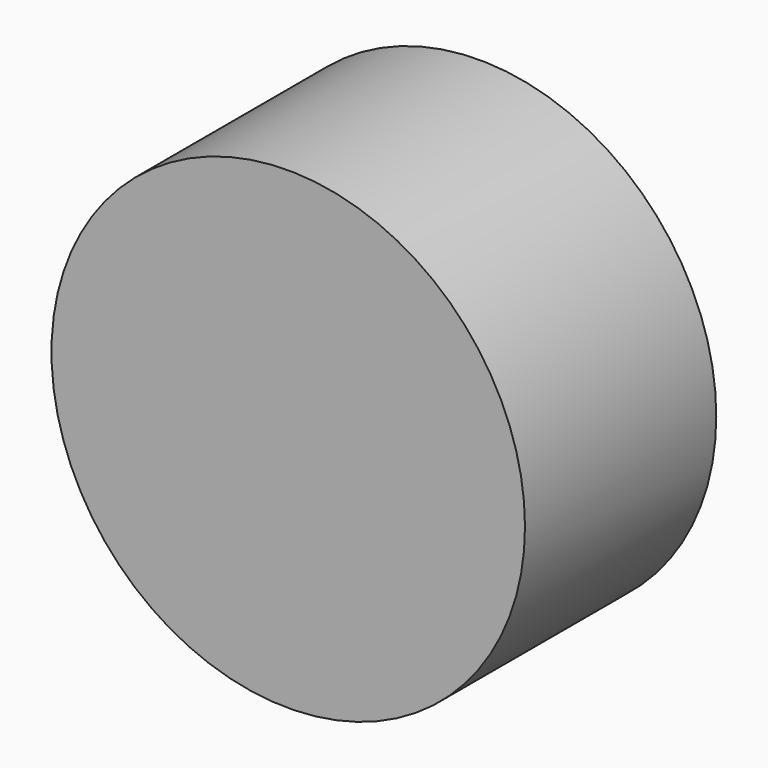
from build123d import *

# Parameters (mm, degrees)
F0_R     = 43.0479033165
F1_DEPTH = 43.4720292687


# Not quite as in the source:
# - the program builds the solid bodies; features that only make, move or delete a surface that nothing else refers to are left out


with BuildPart() as f1:
    # F0 (on Front) → F1 (new body)
    with BuildSketch(Plane.XZ):
        Circle(F0_R)
    extrude(amount=F1_DEPTH)


solid = f1.part
